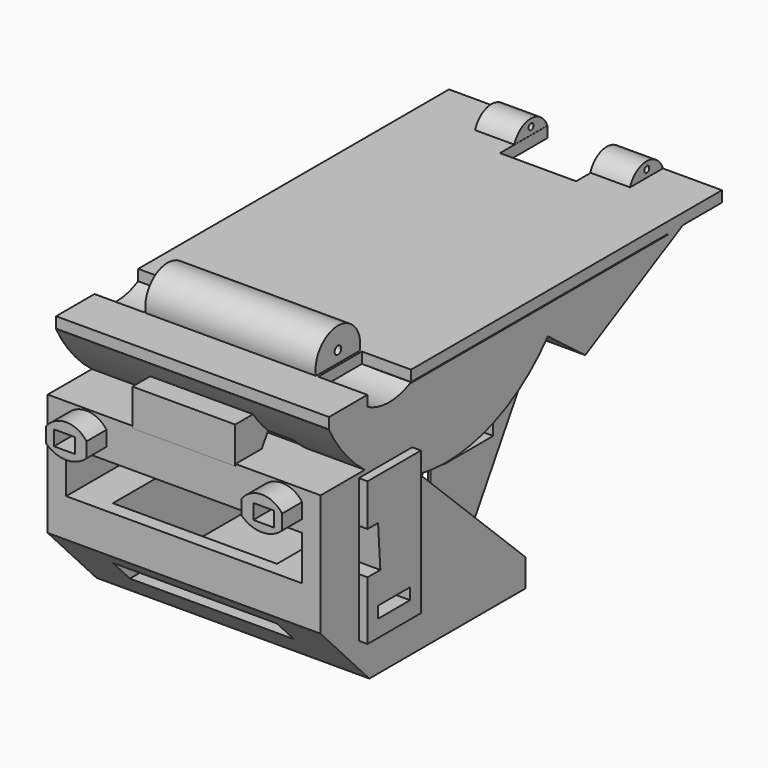
from build123d import *

# Parameters (mm, degrees)
F1_DEPTH  = 1
F2_R      = 0.3763941817
F3_DEPTH  = 7.8
F4_R      = 0.2849523323
F5_DEPTH  = 7.1
F6_W      = 6.9625407923
F6_H      = 3.7631727755
F7_DEPTH  = 25
F10_DEPTH = 12.5
F11_DEPTH = 16.2
F12_W     = 5.614629481
F12_H     = 5.1323007792
F13_DEPTH = 7.3
F15_DEPTH = 23.5
F16_W     = 5.2726729773
F16_H     = 3.5087168217
F17_DEPTH = 25
F19_DEPTH = 14.63
F20_W     = 12.5575540587
F20_H     = 3.0011637136
F21_DEPTH = 14.1
F23_DEPTH = 12.5
F24_W     = 21.6271542013
F24_H     = 4.0732771158
F25_DEPTH = 18
F26_W     = 15.0391664356
F26_H     = 17.8300645202
F27_DEPTH = 14.4
F28_W     = 23.4572906047
F28_H     = 5.0619095564
F29_DEPTH = 25
F31_DEPTH = 25
F32_W     = 0.7207950132
F32_H     = 1.3715437373
F32_W_2   = 1.0647341501
F33_DEPTH = 2.3
F35_DEPTH = 25
F36_DEPTH = 3.9
F37_W     = 3.6760009825
F37_H     = 1.0543689132
F38_DEPTH = 0.8
F39_DEPTH = 3.14


# Not quite as in the source:
# - a feature names something its author has since deleted; it is built from what else it names


with BuildPart() as f1:
    # F0 (on Top) → F1 (new body)
    with BuildSketch(Plane.XY):
        Polygon((-12.5, -22.5), (12.5, -22.5), (12.5, -18.1012732163), (8, -18.1012732163), (8, -13.1012732163), (12.5, -13.1012732163), (12.5, 13.1012732163), (12.5, 18.1012732163), (12.5, 22.5), (3.4913797863, 22.5), (3.4913797863, 17.0689653605), (-3.4913797863, 17.0689653605), (-3.4913797863, 22.5), (-12.5, 22.5), (-12.5, 18.1012732163), (-12.5, 13.1012732163), (-12.5, -13.1012732163), (-8, -13.1012732163), (-8, -18.1012732163), (-12.5, -18.1012732163), align=None)
    extrude(amount=F1_DEPTH)

    # F2 (on Right) → F3 (join, symmetric)
    with BuildSketch(Plane.YZ):
        with BuildLine():
            ThreePointArc((-13.0926464135, 0.9749073963), (-15.5881297193, 4.0409070381), (-18.1252352345, 1.0092595755))
            Line((-18.1252352345, 1.0092595755), (-13.0926464135, 0.9749073963))
        make_face()
        with Locations((-15.6000182033, 2.0549099427)):
            Circle(F2_R, mode=Mode.SUBTRACT)
    extrude(amount=F3_DEPTH, both=True)

    # F8 (on Right) → F10 (join, symmetric)
    with BuildSketch(Plane.YZ):
        with BuildLine():
            Line((6.8501140922, -5.942299962), (18.0227998644, 0))
            Line((18.0227998644, 0), (0, 0))
            Line((0, 0), (-22.5260723382, 0))
            ThreePointArc((-22.5260723382, 0), (-10.6940507845, -8.0376248304), (2.5686097797, -2.6802017819))
            Line((2.5686097797, -2.6802017819), (6.8501140922, -5.942299962))
        make_face()
    extrude(amount=F10_DEPTH, both=True)

    # F9 (on Front) → F11 (join, symmetric)
    with BuildSketch(Plane.XZ):
        with BuildLine():
            Line((12.5918546692, 0), (-12.4535346404, 0))
            ThreePointArc((-12.4535346404, 0), (0.0691600144, -3.8574504381), (12.5918546692, 0))
        make_face()
    extrude(amount=F11_DEPTH, both=True)

    # F12 (on Right) → F13 (join, symmetric)
    with BuildSketch(Plane.YZ):
        Polygon((0, -19.4284636527), (11.7186475545, 0), (-11.9277024642, -8.0778570846), align=None)
        with Locations((0, -9.9393445998)):
            Rectangle(F12_W, F12_H, mode=Mode.SUBTRACT)
    extrude(amount=F13_DEPTH, both=True)

    # F14 (on Front) → F15 (join)
    with BuildSketch(Plane.XZ):
        Polygon((2.2125227842, -5.0941300578), (4.7088093124, -5.0941300578), (4.7088093124, -1.7338488251), align=None)
        Polygon((-2.3142816499, -5.0941300578), (2.2125227842, -5.0941300578), (0, -3.4139894415), align=None)
        Polygon((0, -3.4139894415), (2.2125227842, -5.0941300578), (4.7088093124, -1.7338488251), (-4.7088093124, -1.7338488251), (-2.3142816499, -5.0941300578), align=None)
        Polygon((-4.7088093124, -5.0941300578), (-2.3142816499, -5.0941300578), (-4.7088093124, -1.7338488251), align=None)
    extrude(amount=F15_DEPTH)

    # F16 (on face) → F17 (cut)
    with BuildSketch(Plane(origin=(0, 8.5925626224, -5.1827676527), x_dir=(-1, 0, 0), z_dir=(0, 0.8562934196, -0.5164896703))):
        with Locations((4.4602244161, -13.1185930222)):
            Rectangle(F16_W, F16_H)
        with Locations((-4.4602244161, -13.1185930222)):
            Rectangle(F16_W, F16_H)
    extrude(amount=-F17_DEPTH, mode=Mode.SUBTRACT)

    # F18 (on Right) → F19 (cut, symmetric)
    with BuildSketch(Plane.YZ):
        with BuildLine():
            Line((-13.1277358159, 0), (-18.0616602302, 0))
            ThreePointArc((-18.0616602302, 0), (-15.5946980231, -0.6176502796), (-13.1277358159, 0))
        make_face()
    extrude(amount=F19_DEPTH, both=True, mode=Mode.SUBTRACT)

    # F20 (on face) → F21 (cut)
    with BuildSketch(Plane(origin=(0, 8.5925626224, -5.1827676527), x_dir=(-1, 0, 0), z_dir=(0, 0.8562934196, -0.5164896703))):
        with Locations((0, -7.2315600701)):
            Rectangle(F20_W, F20_H)
    extrude(amount=-F21_DEPTH, mode=Mode.SUBTRACT)

    # F22 (on Right) → F23 (join, symmetric)
    with BuildSketch(Plane.YZ):
        Polygon((-23.4572906047, -19.445579499), (0, -19.445579499), (-12.1369604021, -7.8257964924), (-18.2801373303, -4.9292426556), (-23.4572906047, -4.9292426556), align=None)
    extrude(amount=F23_DEPTH, both=True)

    # F24 (on face) → F25 (cut)
    with BuildSketch(Plane.XZ.offset(23.4572906047)):
        with Locations((0, -10.5389403179)):
            Rectangle(F24_W, F24_H)
    extrude(amount=-F25_DEPTH, mode=Mode.SUBTRACT)

    # F26 (on face) → F27 (cut)
    with BuildSketch(Plane(origin=(0, 0, -19.445579499), x_dir=(1, 0, 0), z_dir=(0, 0, -1))):
        with Locations((0, 13.3097972721)):
            Rectangle(F26_W, F26_H)
    extrude(amount=-F27_DEPTH, mode=Mode.SUBTRACT)

    # F28 (on face) → F29 (join)
    with BuildSketch(Plane.YZ.offset(12.5)):
        with Locations((-11.7286453024, -21.9765342772)):
            Rectangle(F28_W, F28_H)
    extrude(amount=-F29_DEPTH)

    # F30 (on face) → F31 (cut)
    with BuildSketch(Plane(origin=(-12.5, 0, 0), x_dir=(0, -1, 0), z_dir=(-1, 0, 0))):
        Polygon((23.4572906047, -16.9349499047), (23.4572906047, -16.0875618458), (15.4805742204, -24.5074890554), (23.4572906047, -24.5074890554), align=None)
    extrude(amount=-F31_DEPTH, mode=Mode.SUBTRACT)

    # F32 (on face) → F33 (join)
    with BuildSketch(Plane.XZ.offset(23.4572906047)):
        with BuildLine():
            ThreePointArc((-7.1081467904, -6.0146130861), (-8.9597303886, -5.0757459096), (-10.8113139868, -6.0146130861))
            Line((-10.8113139868, -6.0146130861), (-10.0905189736, -6.0146130861))
            Line((-10.0905189736, -6.0146130861), (-8.1728809406, -6.0146130861))
            Line((-8.1728809406, -6.0146130861), (-7.1081467904, -6.0146130861))
        make_face()
        with Locations((-10.4509164802, -6.7003849548)):
            Rectangle(F32_W, F32_H)
        with BuildLine():
            Line((-10.0905189736, -7.3861568235), (-10.8113139868, -7.3861568235))
            ThreePointArc((-10.8113139868, -7.3861568235), (-10.4708156825, -7.6599212202), (-10.0905189736, -7.8750036537))
            Line((-10.0905189736, -7.8750036537), (-10.0905189736, -7.3861568235))
        make_face()
        with Locations((-7.6405138655, -6.7003849548)):
            Rectangle(F32_W_2, F32_H)
        Polygon((-8.1728809406, -7.3861568235), (-10.0905189736, -7.3861568235), (-10.0905189736, -7.8750036537), (-8.1728809406, -8.0064474552), align=None)
        with BuildLine():
            Line((-8.1728809406, -8.0064474552), (-10.0905189736, -7.8750036537))
            ThreePointArc((-10.0905189736, -7.8750036537), (-9.143830635, -8.1177004217), (-8.1728809406, -8.0064474552))
        make_face()
        with BuildLine():
            ThreePointArc((-8.1728809406, -8.0064474552), (-7.6045468764, -7.7580397823), (-7.1081467904, -7.3861568235))
            Line((-7.1081467904, -7.3861568235), (-8.1728809406, -7.3861568235))
            Line((-8.1728809406, -7.3861568235), (-8.1728809406, -8.0064474552))
        make_face()
        with Locations((10.4509164802, -6.7003849548)):
            Rectangle(F32_W, F32_H)
        with BuildLine():
            Line((10.0905189736, -6.0146130861), (10.8113139868, -6.0146130861))
            ThreePointArc((10.8113139868, -6.0146130861), (8.9597303886, -5.4318557463), (7.1081467904, -6.0146130861))
            Line((7.1081467904, -6.0146130861), (8.1728809406, -6.0146130861))
            Line((8.1728809406, -6.0146130861), (10.0905189736, -6.0146130861))
        make_face()
        with BuildLine():
            ThreePointArc((7.1081467904, -6.0146130861), (8.9597303886, -5.4318557463), (10.8113139868, -6.0146130861))
            ThreePointArc((10.8113139868, -6.0146130861), (8.9597303886, -5.0757459096), (7.1081467904, -6.0146130861))
        make_face()
        with BuildLine():
            ThreePointArc((10.0905189736, -7.8750036537), (10.4708156825, -7.6599212202), (10.8113139868, -7.3861568235))
            Line((10.8113139868, -7.3861568235), (10.0905189736, -7.3861568235))
            Line((10.0905189736, -7.3861568235), (10.0905189736, -7.8750036537))
        make_face()
        with Locations((7.6405138655, -6.7003849548)):
            Rectangle(F32_W_2, F32_H)
        Polygon((10.0905189736, -7.8750036537), (10.0905189736, -7.3861568235), (8.1728809406, -7.3861568235), (8.1728809406, -8.0064474552), align=None)
        with BuildLine():
            ThreePointArc((8.1728809406, -8.0064474552), (9.143830635, -8.1177004217), (10.0905189736, -7.8750036537))
            Line((10.0905189736, -7.8750036537), (8.1728809406, -8.0064474552))
        make_face()
        with BuildLine():
            Line((8.1728809406, -7.3861568235), (7.1081467904, -7.3861568235))
            ThreePointArc((7.1081467904, -7.3861568235), (7.6045468764, -7.7580397823), (8.1728809406, -8.0064474552))
            Line((8.1728809406, -8.0064474552), (8.1728809406, -7.3861568235))
        make_face()
    extrude(amount=F33_DEPTH)

    # F34 (on face) → F35 (cut)
    with BuildSketch(Plane.YZ.offset(12.5)):
        Polygon((-17.8783037903, -21.9765342772), (-15.4805742204, -24.5074890554), (0, -24.5074890554), (0, -21.9765342772), (-15.4805742204, -21.9765342772), align=None)
    extrude(amount=-F35_DEPTH, mode=Mode.SUBTRACT)

    # F34 (on face) → F36 (cut)
    with BuildSketch(Plane.YZ.offset(12.5)):
        Polygon((-17.8783037903, -21.9765342772), (-15.4805742204, -24.5074890554), (0, -24.5074890554), (0, -21.9765342772), (-15.4805742204, -21.9765342772), align=None)
    extrude(amount=F36_DEPTH, mode=Mode.SUBTRACT)

    # F37 (on face) → F38 (join)
    with BuildSketch(Plane.YZ.offset(12.5)):
        Polygon((-18.4822846204, -6.4001819119), (-18.4822846204, -9.1605170985), (-17.8783037903, -9.1605170985), (-17.6186137279, -13.0569394678), (-18.4822846204, -13.0569394678), (-18.4822846204, -17.3515146598), (-13.5730896145, -17.3515146598), (-13.5730896145, -6.4001819119), align=None)
        with Locations((-16.0463098437, -16.36005193)):
            Rectangle(F37_W, F37_H, mode=Mode.SUBTRACT)
        Polygon((-12.9706393927, -5.3143799305), (-19.0847348422, -5.3143799305), (-19.0847348422, -9.1605170985), (-18.4822846204, -9.1605170985), (-18.4822846204, -6.4001819119), (-13.5730896145, -6.4001819119), (-13.5730896145, -17.3515146598), (-18.4822846204, -17.3515146598), (-18.4822846204, -13.0569394678), (-19.0847348422, -13.0569394678), (-19.0847348422, -18.4373166412), (-12.9706393927, -18.4373166412), align=None)
    extrude(amount=F38_DEPTH)

    # F37 (on face) → F39 (cut)
    with BuildSketch(Plane.YZ.offset(12.5)):
        Polygon((-18.4822846204, -9.1605170985), (-19.0847348422, -9.1605170985), (-19.0847348422, -13.0569394678), (-18.4822846204, -13.0569394678), (-17.6186137279, -13.0569394678), (-17.8783037903, -9.1605170985), align=None)
        with Locations((-16.0463098437, -16.36005193)):
            Rectangle(F37_W, F37_H)
    extrude(amount=-F39_DEPTH, mode=Mode.SUBTRACT)


with BuildPart() as f5:
    # F4 (on Right) → F5 (new body, symmetric)
    with BuildSketch(Plane.YZ):
        with BuildLine():
            Line((18.7312345952, 1.0029911064), (22.4944073707, 1.0029911064))
            ThreePointArc((22.4944073707, 1.0029911064), (20.6128209829, 2.3433464881), (18.7312345952, 1.0029911064))
        make_face()
        with Locations((20.642824471, 1.6716184327)):
            Circle(F4_R, mode=Mode.SUBTRACT)
    extrude(amount=F5_DEPTH, both=True)

    # F6 (on face) → F7 (cut)
    with BuildSketch(Plane(origin=(0, 0, 1.0029911064), x_dir=(1, 0, 0), z_dir=(0, 0, -1))):
        with Locations((-0.0190356513, -20.6128209829)):
            Rectangle(F6_W, F6_H)
    extrude(amount=-F7_DEPTH, mode=Mode.SUBTRACT)


solid = Compound([f1.part, f5.part])
